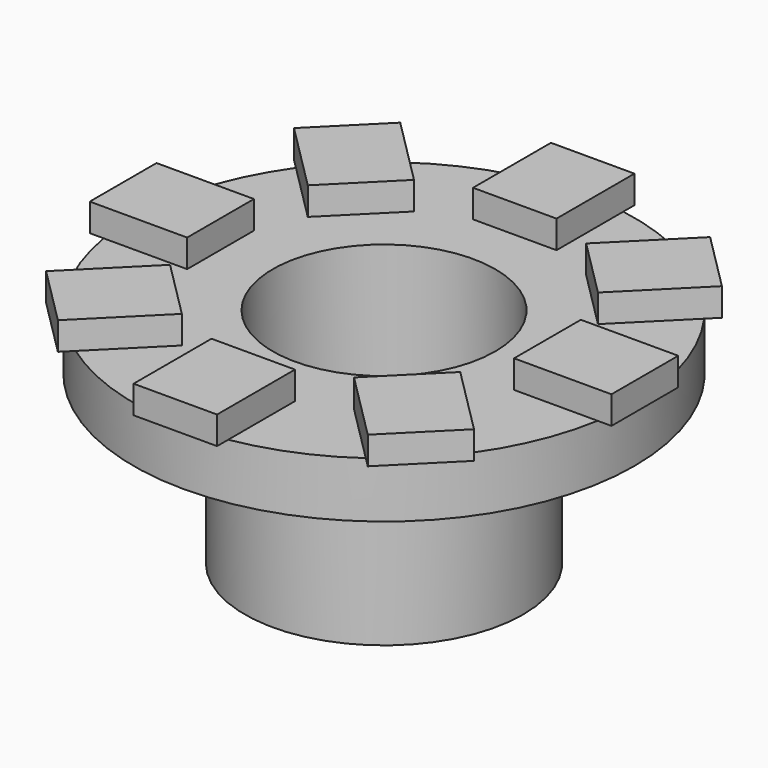
from build123d import *

# Parameters (mm, degrees)
F4_DEPTH = 6.35
F5_COUNT = 8


# Not quite as in the source:
# - a feature names something its author has since deleted; it is built from what else it names


with BuildPart() as f1:
    # F0 (on Front) → F1 (revolve)
    with BuildSketch(Plane.XZ):
        Polygon((25.4, 0), (25.4, -50.8), (31.75, -50.8), (31.75, -12.7), (57.15, -12.7), (57.15, 0), align=None)
    revolve(axis=Axis((0, 0, 2.673143521), (0, 0, -1)))

    # F2 (on face) → F4 (join)
    with BuildSketch(Plane.XY):
        with BuildLine():
            ThreePointArc((57.15, 0), (56.9498143774, -4.779240775), (56.350659934, -9.525))
            Line((56.350659934, -9.525), (59.525659934, -9.525))
            Line((59.525659934, -9.525), (59.525659934, 9.525))
            Line((59.525659934, 9.525), (56.350659934, 9.525))
            ThreePointArc((56.350659934, 9.525), (56.9498143774, 4.779240775), (57.15, 0))
        make_face()
        with BuildLine():
            Line((37.300659934, 9.525), (37.300659934, -9.525))
            Line((37.300659934, -9.525), (56.350659934, -9.525))
            ThreePointArc((56.350659934, -9.525), (56.9498143774, -4.779240775), (57.15, 0))
            ThreePointArc((57.15, 0), (56.9498143774, 4.779240775), (56.350659934, 9.525))
            Line((56.350659934, 9.525), (37.300659934, 9.525))
        make_face()
    extrude(amount=F4_DEPTH)

    # F5: F1 ×8 about axis
    f5_axis = Axis((0, 0, 22.2758), (0, 0, 1))


with BuildPart() as f1_1:
    add(f1.part)
    for i in range(1, F5_COUNT):
        add(f1.part.rotate(f5_axis, i * 360 / F5_COUNT))


solid = f1_1.part
